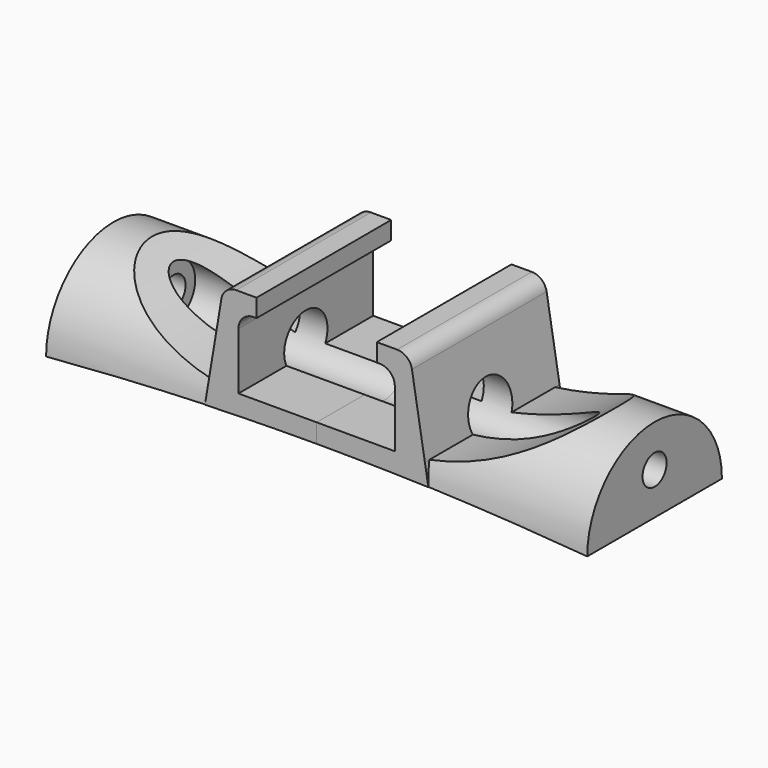
from build123d import *

# Parameters (mm, degrees)
F1_DEPTH = 28
F2_R     = 2.5
F3_REACH = 79.4103010682
F4_R     = 4.5
F5_DEPTH = 35


with BuildPart() as f1:
    # F0 (on Front) → F1 (new body)
    with BuildSketch(Plane.XZ):
        with BuildLine():
            ThreePointArc((0, 1.8460551577), (22.518924928, 1.3843473584), (45, 0))
            Line((45, 0), (45, 20))
            ThreePointArc((45, 20), (32.777940188, 10.1997076616), (18, 5))
            Line((18, 5), (15.8481670886, 17.9109974683))
            ThreePointArc((15.8481670886, 17.9109974683), (14.9981195194, 19.4075499562), (13.382182279, 20))
            Line((13.382182279, 20), (10, 20))
            Line((10, 20), (10, 17))
            Line((10, 17), (10.5, 17))
            ThreePointArc((10.5, 17), (12.267766953, 16.267766953), (13, 14.5))
            Line((13, 14.5), (13, 5))
            Line((13, 5), (0, 5))
            Line((0, 5), (0, 1.8460551577))
        make_face()
    extrude(amount=F1_DEPTH)

    f3_end = Plane(origin=(16.9240835443, -14, 11.4554987341), x_dir=(-0.1643989873, 0, 0.9863939238), z_dir=(0.9863939238, 0, 0.1643989873))
    # F2 (on face) → F3 (cut, up to a plane its end follows)
    with BuildSketch(Plane.YZ.offset(45)):
        with BuildLine():
            ThreePointArc((-28, 0), (-14, 14), (0, 0))
            Line((0, 0), (0, 20))
            Line((0, 20), (-28, 20))
            Line((-28, 20), (-28, 0))
        make_face()
        with Locations((-14, 7)):
            Circle(F2_R)
    f3_long = extrude(amount=-F3_REACH, mode=Mode.PRIVATE)
    add(split(f3_long, bisect_by=f3_end, keep=Keep.TOP, mode=Mode.PRIVATE), mode=Mode.SUBTRACT)

    # F4 (on face) → F5 (cut)
    with BuildSketch(Plane(origin=(0, 0, 0), x_dir=(0, -1, 0), z_dir=(-1, 0, 0))):
        with Locations((14.0023827553, 7)):
            Circle(F4_R)
    extrude(amount=-F5_DEPTH, mode=Mode.SUBTRACT)


with BuildPart() as f6_1:
    # F6: instance of F1
    add(f1.part.mirror(Plane(origin=(0, -13.9995349906, 3.3159781589), x_dir=(0, -1, 0), z_dir=(-1, 0, 0))))


solid = Compound([f1.part, f6_1.part])
